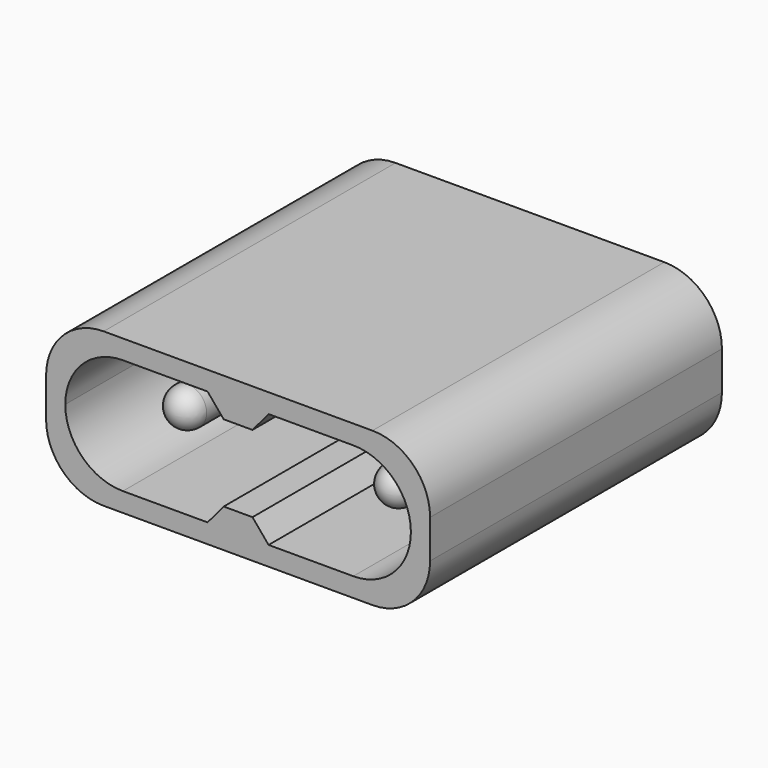
from build123d import *

# Parameters (mm, degrees)
F1_DEPTH = 17
F2_R     = 1
F3_DEPTH = 15
F4_R     = 1
F4_2_R   = 1
F6_DEPTH = 2
F8_DEPTH = 0.1


with BuildPart() as f1:
    # F0 (on Front) → F1 (new body)
    with BuildSketch(Plane.XZ):
        with BuildLine():
            ThreePointArc((10, 1), (9.1213203436, 3.1213203436), (7, 4))
            Line((7, 4), (-7, 4))
            ThreePointArc((-7, 4), (-9.1213203436, 3.1213203436), (-10, 1))
            Line((-10, 1), (-10, -1))
            ThreePointArc((-10, -1), (-9.1213203436, -3.1213203436), (-7, -4))
            Line((-7, -4), (7, -4))
            ThreePointArc((7, -4), (9.1213203436, -3.1213203436), (10, -1))
            Line((10, -1), (10, 1))
        make_face()
        with BuildLine():
            ThreePointArc((-9, 0), (-8.1213203436, 2.1213203436), (-6, 3))
            Line((-6, 3), (-1.5890996312, 3))
            Line((-1.5890996312, 3), (-0.75, 2))
            Line((-0.75, 2), (0, 2))
            Line((0, 2), (0.75, 2))
            Line((0.75, 2), (1.5890996312, 3))
            Line((1.5890996312, 3), (6, 3))
            ThreePointArc((6, 3), (8.1213203436, 2.1213203436), (9, 0))
            ThreePointArc((9, 0), (8.1213203436, -2.1213203436), (6, -3))
            Line((6, -3), (1.5890996312, -3))
            Line((1.5890996312, -3), (0.75, -2))
            Line((0.75, -2), (0, -2))
            Line((0, -2), (-0.75, -2))
            Line((-0.75, -2), (-1.5890996312, -3))
            Line((-1.5890996312, -3), (-6, -3))
            ThreePointArc((-6, -3), (-8.1213203436, -2.1213203436), (-9, 0))
        make_face(mode=Mode.SUBTRACT)
    extrude(amount=F1_DEPTH)

    # F5 (on face) → F6 (join)
    with BuildSketch(Plane.XZ):
        with BuildLine():
            ThreePointArc((10, 1), (9.1213203436, 3.1213203436), (7, 4))
            Line((7, 4), (-7, 4))
            ThreePointArc((-7, 4), (-9.1213203436, 3.1213203436), (-10, 1))
            Line((-10, 1), (-10, -1))
            ThreePointArc((-10, -1), (-9.1213203436, -3.1213203436), (-7, -4))
            Line((-7, -4), (7, -4))
            ThreePointArc((7, -4), (9.1213203436, -3.1213203436), (10, -1))
            Line((10, -1), (10, 1))
        make_face()
    extrude(amount=-F6_DEPTH)


with BuildPart() as f3:
    # F2 (on Front) → F3 (new body)
    with BuildSketch(Plane.XZ):
        with Locations((-5.0379058985, 0)):
            Circle(F2_R)
    extrude(amount=F3_DEPTH)

    # F4
    f4_edges = [f3.edges().sort_by_distance(p)[0] for p in [
        (-6.037906, -15, 0),
    ]]
    fillet(f4_edges, radius=F4_R)



with BuildPart() as f3b:
    # F2 (on Front) → F3, piece 2 (new body)
    with BuildSketch(Plane.XZ):
        with Locations((5.9620941015, 0)):
            Circle(F2_R)
    extrude(amount=F3_DEPTH)

    # F4#2
    f4_2_edges = [f3b.edges().sort_by_distance(p)[0] for p in [
        (4.962094, -15, 0),
    ]]
    fillet(f4_2_edges, radius=F4_2_R)


with BuildPart() as f3_1:
    add(f3.part)

    add(f3b.part)  # F8 merges F3b
    # F7 (on face) → F8 (join)
    with BuildSketch(Plane.XZ):
        with BuildLine():
            Line((-0.75, 2), (-1.5890996312, 3))
            Line((-1.5890996312, 3), (-6, 3))
            ThreePointArc((-6, 3), (-9, 0), (-6, -3))
            Line((-6, -3), (-1.5890996312, -3))
            Line((-1.5890996312, -3), (-0.75, -2))
            Line((-0.75, -2), (0.75, -2))
            Line((0.75, -2), (1.5890996312, -3))
            Line((1.5890996312, -3), (6, -3))
            ThreePointArc((6, -3), (9, 0), (6, 3))
            Line((6, 3), (1.5890996312, 3))
            Line((1.5890996312, 3), (0.75, 2))
            Line((0.75, 2), (-0.75, 2))
        make_face()
    extrude(amount=F8_DEPTH)


solid = Compound([f1.part, f3_1.part])
